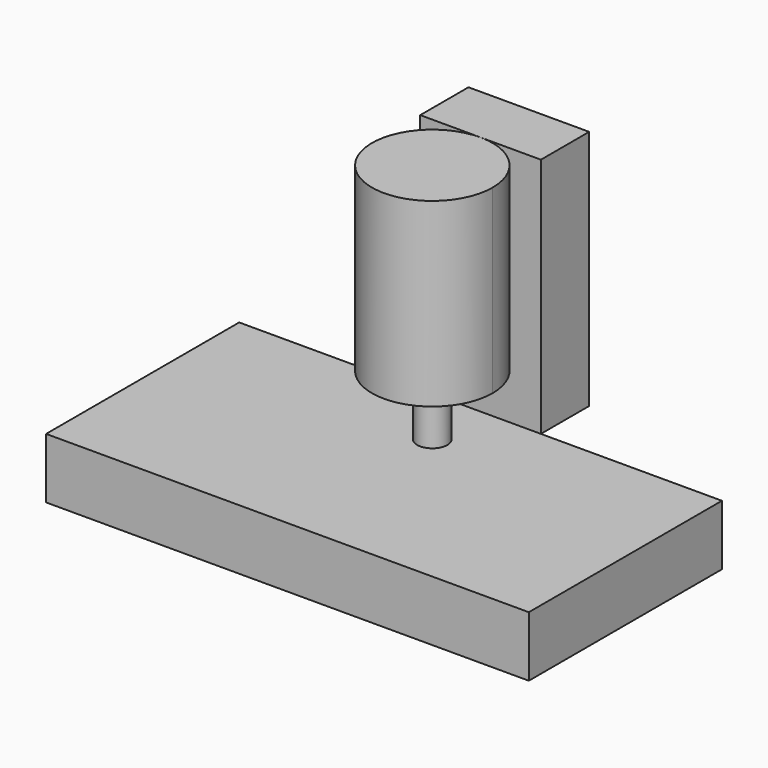
from build123d import *

# Parameters (mm, degrees)
F0_W     = 101.6
F0_H     = 50.8
F1_DEPTH = 12.7
F2_W     = 25.4
F2_H     = 50.8
F3_DEPTH = 12.7
F5_DEPTH = 38.1
F6_R     = 3.175
F7_DEPTH = 12.7


with BuildPart() as f1:
    # F0 (on Top) → F1 (new body)
    with BuildSketch(Plane.XY):
        Rectangle(F0_W, F0_H)
    extrude(amount=F1_DEPTH)


with BuildPart() as f3:
    # F2 (on face) → F3 (new body)
    with BuildSketch(Plane(origin=(0, 25.4, 0), x_dir=(-1, 0, 0), z_dir=(0, 1, 0))):
        with Locations((0, 38.1)):
            Rectangle(F2_W, F2_H)
    extrude(amount=F3_DEPTH)


with BuildPart() as f5:
    # F4 (on face) → F5 (new body)
    with BuildSketch(Plane.XY.offset(63.5)):
        with BuildLine():
            ThreePointArc((1.16e-08, 25.4), (-8.9802561252, 3.719743883), (12.7, 12.7))
            ThreePointArc((12.7, 12.7), (8.9802561252, 21.680256117), (1.16e-08, 25.4))
        make_face()
    extrude(amount=-F5_DEPTH)

    # F6 (on face) → F7 (join)
    with BuildSketch(Plane(origin=(0, 0, 25.4), x_dir=(1, 0, 0), z_dir=(0, 0, -1))):
        with Locations((0, -12.7)):
            Circle(F6_R)
    extrude(amount=F7_DEPTH)


solid = Compound([f1.part, f3.part, f5.part])
